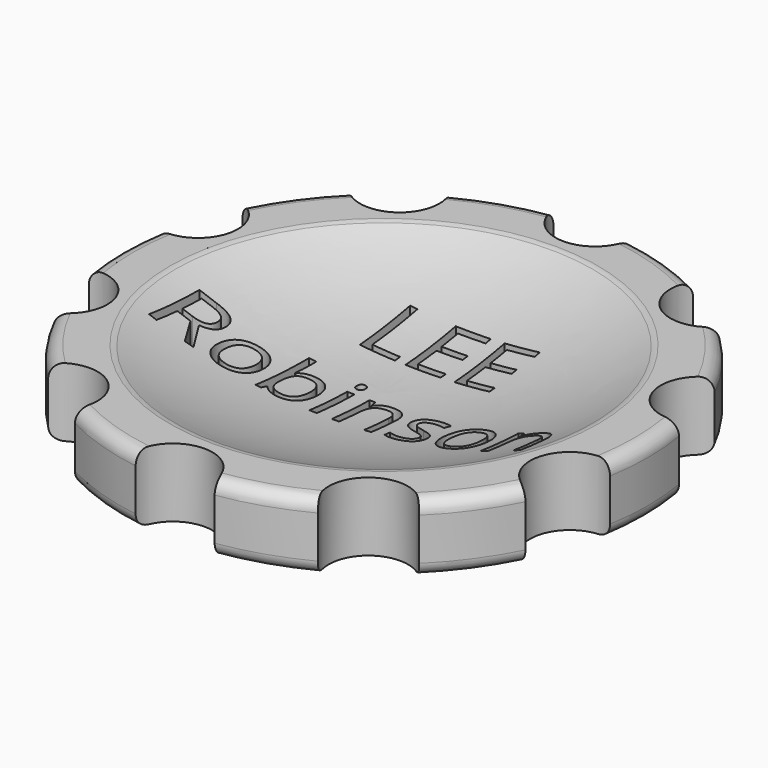
from build123d import *

# Parameters (mm, degrees)
F2_R         = 7.5
F3_DEPTH     = 13.018514788
F5_COUNT     = 10
F6_TEXT_SIZE = 16.6666666667
F8_DEPTH     = 25
F7_TEXT_SIZE = 16.6666666667
F9_DEPTH     = 25
F10_W        = 9.892705828
F10_H        = 2.810427919
F11_DEPTH    = 3
F10_W_2      = 9.3306237832
F10_H_2      = 2.922845073
F10_W_3      = 9.5554515719
F10_W_4      = 10.3423781693
F10_H_3      = 2.0235083066


# Not quite as in the source:
# - Text() gives the source's letters only with a copy of the font that has no kerning and outlines rounded to 1/6400 em; it was checked with that copy


with BuildPart() as f1:
    # F0 (on Front) → F1 (revolve)
    with BuildSketch(Plane.XZ):
        with BuildLine():
            Line((-47.5, 0), (0, 0))
            Line((0, 0), (0, 5))
            ThreePointArc((0, 5), (-20.1939988569, 6.7061448874), (-39.5207867833, 12.8039960382))
            ThreePointArc((-39.5207867833, 12.8039960382), (-40.0151065255, 12.9635527196), (-40.5317286671, 13.017514788))
            Line((-40.5317286671, 13.017514788), (-47.5, 13.017514788))
            ThreePointArc((-47.5, 13.017514788), (-49.267766953, 12.2852817409), (-50, 10.517514788))
            Line((-50, 10.517514788), (-50, 2.5))
            ThreePointArc((-50, 2.5), (-49.267766953, 0.732233047), (-47.5, 0))
        make_face()
    revolve(axis=Axis((0, 0, 2.5), (0, 0, 1)))

    # F2 (on Top) → F3 (cut, through all)
    with BuildSketch(Plane.XY):
        with Locations((0, -49.9895140529)):
            Circle(F2_R)
    f3 = extrude(amount=F3_DEPTH, mode=Mode.SUBTRACT)

    # F5: F3 ×10 about axis
    f5_axis = Axis((0, 0, 20.1124101877), (0, 0, -1))
    for i in range(1, F5_COUNT):
        add(f3.rotate(f5_axis, i * 360 / F5_COUNT), mode=Mode.SUBTRACT)

    # F6 (on Top) → F8 (cut)
    with BuildSketch(Plane.XY):
        with Locations((-13.1764722871, 8.7058850226)):
            Text('LEE', F6_TEXT_SIZE, font='Open Sans', text_align=(TextAlign.LEFT, TextAlign.BOTTOM))
    extrude(amount=F8_DEPTH, mode=Mode.SUBTRACT)

    # F7 (on Top) → F9 (cut)
    with BuildSketch(Plane.XY):
        with Locations((-36.5078125, -12)):
            Text('Robinson', F7_TEXT_SIZE, font='Open Sans', text_align=(TextAlign.LEFT, TextAlign.BOTTOM))
    extrude(amount=F9_DEPTH, mode=Mode.SUBTRACT)


with BuildPart() as f11:
    # F10 (on Top) → F11 (new body)
    with BuildSketch(Plane.XY):
        with Locations((21.6273684055, -7.5381947681)):
            Rectangle(F10_W, F10_H)
    extrude(amount=F11_DEPTH)


with BuildPart() as f11b:
    # F10 (on Top) → F11, piece 2 (new body)
    with BuildSketch(Plane.XY):
        with Locations((-10.8049712144, -7.4819861911)):
            Rectangle(F10_W_2, F10_H_2)
    extrude(amount=F11_DEPTH)


with BuildPart() as f11c:
    # F10 (on Top) → F11, piece 3 (new body)
    with BuildSketch(Plane.XY):
        with Locations((-21.3721804321, -7.4819861911)):
            Rectangle(F10_W_3, F10_H_2)
    extrude(amount=F11_DEPTH)


with BuildPart() as f11d:
    # F10 (on Top) → F11, piece 4 (new body)
    with BuildSketch(Plane.XY):
        with Locations((-31.3210953027, -3.3225526568)):
            Rectangle(F10_W_4, F10_H_3)
    extrude(amount=F11_DEPTH)


solid = Compound([f1.part, f11.part, f11b.part, f11c.part, f11d.part])
